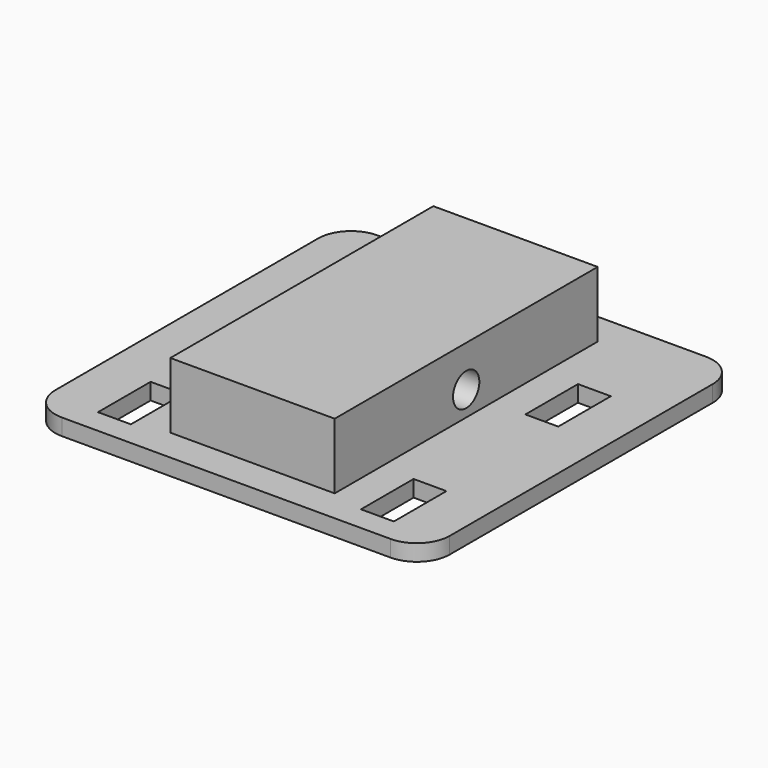
from build123d import *

# Parameters (mm, degrees)
F2_DEPTH = 6.35
F3_W     = 63.5
F3_H     = 127
F4_DEPTH = 25.4
F5_R     = 6.35
F6_DEPTH = 63.5
F7_W     = 12.7
F7_H     = 25.4
F8_DEPTH = 6.35


# Not quite as in the source:
# - the program builds the solid bodies; features that only make, move or delete a surface that nothing else refers to are left out


with BuildPart() as f2:
    # F0 (on Top) → F2 (new body)
    with BuildSketch(Plane.XY):
        with BuildLine():
            Line((63.5, 76.2), (-63.5, 76.2))
            ThreePointArc((-63.5, 76.2), (-72.4802561211, 72.4802561211), (-76.2, 63.5))
            Line((-76.2, 63.5), (-76.2, -63.5))
            ThreePointArc((-76.2, -63.5), (-72.4802561211, -72.4802561211), (-63.5, -76.2))
            Line((-63.5, -76.2), (63.5, -76.2))
            ThreePointArc((63.5, -76.2), (72.4802561211, -72.4802561211), (76.2, -63.5))
            Line((76.2, -63.5), (76.2, 63.5))
            ThreePointArc((76.2, 63.5), (72.4802561211, 72.4802561211), (63.5, 76.2))
        make_face()
        with BuildLine():
            ThreePointArc((-69.85, 57.15), (-66.1302561211, 66.1302561211), (-57.15, 69.85))
            Line((-57.15, 69.85), (-1.846e-07, 69.85))
            Line((-1.846e-07, 69.85), (57.15, 69.85))
            ThreePointArc((57.15, 69.85), (66.1302561211, 66.1302561211), (69.85, 57.15))
            Line((69.85, 57.15), (69.85, 0))
            Line((69.85, 0), (69.85, -57.15))
            ThreePointArc((69.85, -57.15), (66.1302561211, -66.1302561211), (57.15, -69.85))
            Line((57.15, -69.85), (0, -69.85))
            Line((0, -69.85), (-57.15, -69.85))
            ThreePointArc((-57.15, -69.85), (-66.1302561211, -66.1302561211), (-69.85, -57.15))
            Line((-69.85, -57.15), (-69.85, -1.807e-07))
            Line((-69.85, -1.807e-07), (-69.85, 57.15))
        make_face(mode=Mode.SUBTRACT)
        with BuildLine():
            ThreePointArc((69.85, 0), (49.3914086006, 49.3914087312), (-1.846e-07, 69.85))
            ThreePointArc((-1.846e-07, 69.85), (-49.3914087951, 49.3914085367), (-69.85, -1.807e-07))
            ThreePointArc((-69.85, -1.807e-07), (-49.391408602, -49.3914087298), (0, -69.85))
            ThreePointArc((0, -69.85), (49.3914086659, -49.3914086659), (69.85, 0))
        make_face()
        with BuildLine():
            Line((57.15, 69.85), (-1.846e-07, 69.85))
            ThreePointArc((-1.846e-07, 69.85), (49.3914086006, 49.3914087312), (69.85, 0))
            Line((69.85, 0), (69.85, 57.15))
            ThreePointArc((69.85, 57.15), (66.1302561211, 66.1302561211), (57.15, 69.85))
        make_face()
        with BuildLine():
            Line((-1.846e-07, 69.85), (-57.15, 69.85))
            ThreePointArc((-57.15, 69.85), (-66.1302561211, 66.1302561211), (-69.85, 57.15))
            Line((-69.85, 57.15), (-69.85, -1.807e-07))
            ThreePointArc((-69.85, -1.807e-07), (-49.3914087951, 49.3914085367), (-1.846e-07, 69.85))
        make_face()
        with BuildLine():
            Line((69.85, -57.15), (69.85, 0))
            ThreePointArc((69.85, 0), (49.3914086659, -49.3914086659), (0, -69.85))
            Line((0, -69.85), (57.15, -69.85))
            ThreePointArc((57.15, -69.85), (66.1302561211, -66.1302561211), (69.85, -57.15))
        make_face()
        with BuildLine():
            ThreePointArc((0, -69.85), (-49.391408602, -49.3914087298), (-69.85, -1.807e-07))
            Line((-69.85, -1.807e-07), (-69.85, -57.15))
            ThreePointArc((-69.85, -57.15), (-66.1302561211, -66.1302561211), (-57.15, -69.85))
            Line((-57.15, -69.85), (0, -69.85))
        make_face()
    extrude(amount=F2_DEPTH)

    # F3 (on face) → F4 (join)
    with BuildSketch(Plane.XY.offset(6.35)):
        Rectangle(F3_W, F3_H)
    extrude(amount=F4_DEPTH)

    # F5 (on face) → F6 (cut)
    with BuildSketch(Plane.YZ.offset(31.75)):
        with Locations((0, 15.875)):
            Circle(F5_R)
    extrude(amount=-F6_DEPTH, mode=Mode.SUBTRACT)

    # F7 (on face) → F8 (cut)
    with BuildSketch(Plane.XY.offset(6.35)):
        with Locations((50.8, 25.4)):
            Rectangle(F7_W, F7_H)
        with Locations((-50.8, 25.4)):
            Rectangle(F7_W, F7_H)
        with Locations((-50.8, -53.975)):
            Rectangle(F7_W, F7_H)
        with Locations((50.8, -53.975)):
            Rectangle(F7_W, F7_H)
    extrude(amount=-F8_DEPTH, mode=Mode.SUBTRACT)


solid = f2.part
